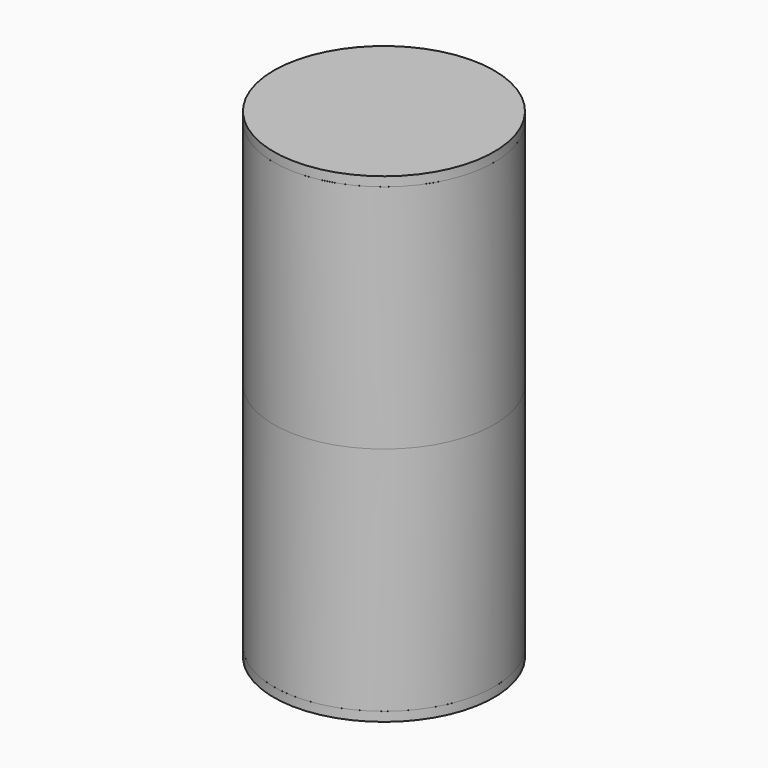
from build123d import *

# Parameters (mm, degrees)
F2_W = 3.5463683307
F2_H = 129.3705441058


with BuildPart() as f1:
    # F0 (on Front) → F1 (revolve)
    with BuildSketch(Plane.XZ):
        Polygon((0, -61.5517236292), (0, -54.612070322), (-58.2384653389, -54.612070322), (-58.2384653389, -56.3352257013), (-61.7407895625, -56.3352257013), (-61.7407895625, -61.5517236292), align=None)
        Polygon((-58.2384653389, -54.612070322), (0, -54.612070322), (0, -52.1982759237), (-12.370692566, -52.1982759237), align=None)
    revolve(axis=Axis((0, 0, -58.0818969756), (0, 0, -1)))


with BuildPart() as f3:
    # F2 (on Front) → F3 (revolve)
    with BuildSketch(Plane.XZ):
        with Locations((-59.9618349224, 8.3581712097)):
            Rectangle(F2_W, F2_H)
    revolve(axis=Axis((0.0027101487, 0, 8.6135864258), (0, 0, 1)))

    # F5: F3 across face


with BuildPart() as f4_1:
    # F4: instance of F1
    add(f1.part.mirror(Plane(origin=(0.0027101487, 0, 73.0434432626), x_dir=(1, 0, 0), z_dir=(0, 0, 1))))


with BuildPart() as f3_1:
    add(f3.part)
    add(f3.part.mirror(Plane(origin=(0.0027101487, 0, 73.0434432626), x_dir=(1, 0, 0), z_dir=(0, 0, 1))))


solid = Compound([f1.part, f4_1.part, f3_1.part])
